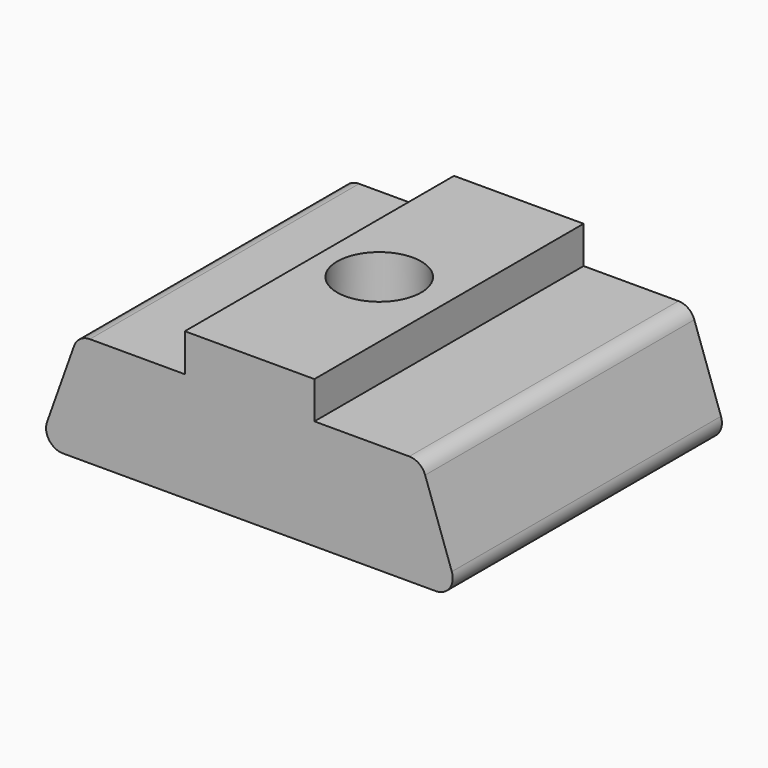
from build123d import *

# Parameters (mm, degrees)
F1_DEPTH = 25.4
F3_D     = 6.35
F4_R     = 3.175
F5_DEPTH = 6.35
F6_R     = 1.27


with BuildPart() as f1:
    # F0 (on Front) → F1 (new body)
    with BuildSketch(Plane.XZ):
        Polygon((-12.6819006406, 8.255), (-15.624309808, 0), (16.125690192, 0), (13.2260993594, 8.3013381809), (5.1634775414, 8.3013381809), (5.1634775414, 11.1125), (-4.6192788226, 11.1125), (-4.6192788226, 8.255), align=None)
    extrude(amount=F1_DEPTH)

    # F3 (through all)
    with Locations(Plane.XY.offset(11.1125)):
        with Locations((0, -12.8323249519)):
            Hole(F3_D / 2)

    # F4 (on face) → F5 (cut)
    with BuildSketch(Plane(origin=(0, 0, 0), x_dir=(1, 0, 0), z_dir=(0, 0, -1))):
        Polygon((-6.4124855846, 13.2020820447), (-3.5264618279, 7.4638280807), (2.8860237566, 7.0940709878), (6.4124855846, 12.462567859), (3.5264618279, 18.2008218231), (-2.8860237566, 18.570578916), align=None)
        with Locations((0, 12.8323249519)):
            Circle(F4_R, mode=Mode.SUBTRACT)
    extrude(amount=-F5_DEPTH, mode=Mode.SUBTRACT)

    # F6
    f6_edges = [f1.edges().sort_by_distance(p)[0] for p in [
        (16.12569, -12.7, 0),
        (-15.62431, -12.7, 0),
        (13.226099, -12.7, 8.301338),
        (-12.681901, -12.7, 8.255),
    ]]
    fillet(f6_edges, radius=F6_R)


solid = f1.part
